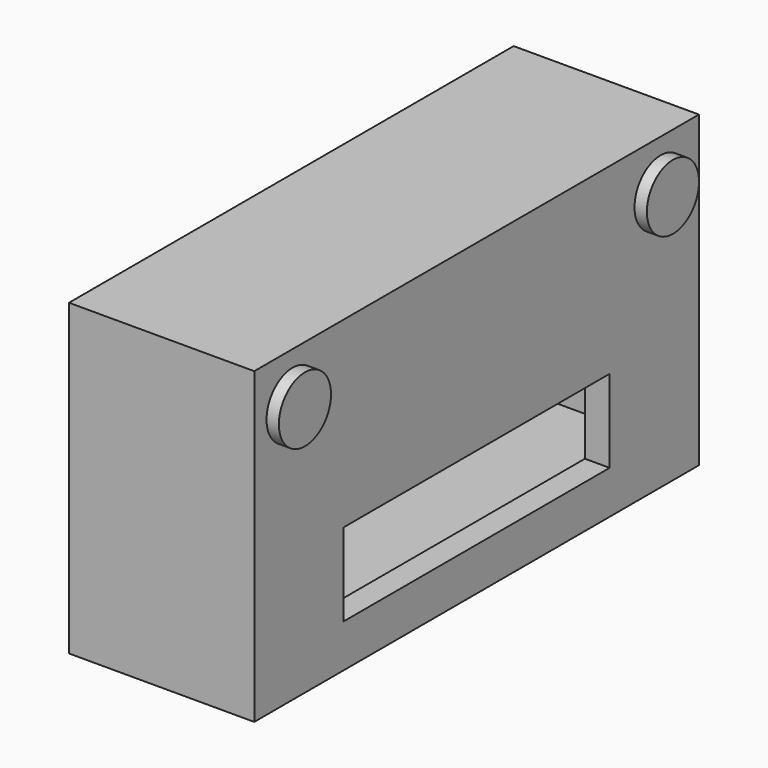
from build123d import *

# Parameters (mm, degrees)
F0_W     = 45
F0_H     = 25
F1_DEPTH = 15
F2_W     = 3.8793105632
F2_H     = 6.7036496475
F2_W_2   = 5.8189658448
F2_W_3   = 7.5361132622
F3_DEPTH = 25
F4_T     = 2
F5_R     = 2.6382169245
F6_DEPTH = 5
F7_DEPTH = 16


# Not quite as in the source:
# - a shell that OpenCascade refuses in one call is made with other operations: the cavity is built on its own and cut out


with BuildPart() as f1:
    # F0 (on Right) → F1 (new body)
    with BuildSketch(Plane.YZ):
        Rectangle(F0_W, F0_H)
    extrude(amount=F1_DEPTH)

    # F2 (on Right) → F3 (join)
    with BuildSketch(Plane.YZ):
        with Locations((-11.5266777575, -5.6595918722)):
            Rectangle(F2_W, F2_H)
        with Locations((-6.6775395535, -5.6595918722)):
            Rectangle(F2_W_2, F2_H)
        with Locations((0, -5.6595918722)):
            Rectangle(F2_W_3, F2_H)
        with Locations((6.6775395535, -5.6595918722)):
            Rectangle(F2_W_2, F2_H)
        with Locations((11.5266777575, -5.6595918722)):
            Rectangle(F2_W, F2_H)
    extrude(amount=F3_DEPTH)

    # F4: shell of thickness 2, made by hand


with BuildPart() as f4_core1:
    # F4_t2: copy of F1
    add(f1.part)

    # the walls: a layer under each face that stays
    f4_faces = [f4_core1.faces().sort_by_distance(p)[0] for p in [
        (7.5, -22.5, 0),
        (7.5, 0, 12.5),
        (7.5, 0, -12.5),
        (0, 0, 0),
        (15, 0, 0),
        (7.5, 22.5, 0),
    ]]
    thicken(f4_faces, amount=-F4_T, mode=Mode.SUBTRACT)


with BuildPart() as f1_1:
    add(f1.part)

    # what is left inside the walls is the cavity
    f4_cavity = [f4_core1.part.solids().sort_by_distance(p)[0] for p in [
        (2.02, 0, -3.5),
    ]]
    add(f4_cavity, mode=Mode.SUBTRACT)

    # F5 (on Right) → F6 (join)
    with BuildSketch(Plane.YZ):
        with Locations((-18.6206903309, 8.5344836116)):
            Circle(F5_R)
        with Locations((18.6206903309, 8.5344836116)):
            Circle(F5_R)
    extrude(amount=F6_DEPTH)

    # F5 (on Right) → F7 (join)
    with BuildSketch(Plane.YZ):
        with Locations((-18.6206903309, 8.5344836116)):
            Circle(F5_R)
        with Locations((18.6206903309, 8.5344836116)):
            Circle(F5_R)
    extrude(amount=F7_DEPTH)


solid = f1_1.part
